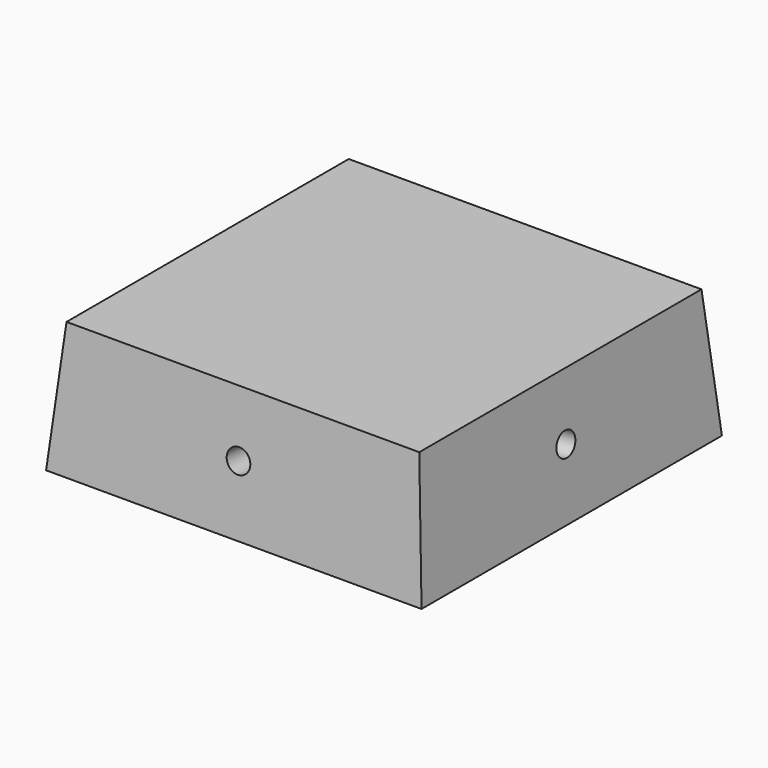
from build123d import *

# Parameters (mm, degrees)
F0_W        = 101.6
F0_H        = 101.6
F1_DEPTH    = 34.925
F2_T1_DEPTH = 299.3404177556
F2_T3_DEPTH = 299.3404177556
F3_R        = 3.175
F4_DEPTH    = 12.7
F5_R        = 3.175
F6_DEPTH    = 12.7
F7_R        = 3.175
F8_DEPTH    = 12.7
F9_R        = 3.175
F10_DEPTH   = 12.7
F11_W       = 75.6562831473
F11_H       = 25.4
F12_DEPTH   = 25.4
F13_SIZE2   = 25.39999
F13_SIZE    = 2.53999
F15_DEPTH   = 12.7
F16_R       = 2.54


# Not quite as in the source:
# - a fillet or chamfer that OpenCascade refuses, or shapes differently, is made with other operations: its cross-section is extruded or revolved along the edge and cut away or added
# - a fillet or chamfer is up to 0.001 mm smaller than in the source, because OpenCascade refuses the exact size


with BuildPart() as f1:
    # F0 (on Top) → F1 (new body)
    with BuildSketch(Plane.XY):
        Rectangle(F0_W, F0_H)
    extrude(amount=F1_DEPTH)

    # F2: chamfer of 3.3274 x 38.0323560322 on 4 edges, made by hand

    # F2_s2 → F2_t1 (cut)
    with BuildSketch(Plane.XZ.offset(-149.6702088778)):
        Polygon((-50.8, -3.1073560322), (-47.4726, 34.925), (-50.8, 34.925), align=None)
        Polygon((50.8, -3.1073560322), (47.4726, 34.925), (50.8, 34.925), align=None)
    extrude(amount=F2_T1_DEPTH, mode=Mode.SUBTRACT)

    # F2_s4 → F2_t3 (cut)
    with BuildSketch(Plane.YZ.offset(-149.6702088778)):
        Polygon((-50.8, -3.1073560322), (-47.4726, 34.925), (-50.8, 34.925), align=None)
        Polygon((50.8, -3.1073560322), (47.4726, 34.925), (50.8, 34.925), align=None)
    extrude(amount=F2_T3_DEPTH, mode=Mode.SUBTRACT)

    # F3 (on face) → F4 (cut)
    with BuildSketch(Plane(origin=(0, 50.1443235703, 4.3870598526), x_dir=(-1, 0, 0), z_dir=(0, 0.9961946981, 0.0871557427))):
        with Locations((0, 13.6719250414)):
            Circle(F3_R)
    extrude(amount=-F4_DEPTH, mode=Mode.SUBTRACT)

    # F5 (on face) → F6 (cut)
    with BuildSketch(Plane(origin=(0, -50.1443235703, 4.3870598526), x_dir=(1, 0, 0), z_dir=(0, -0.9961946981, 0.0871557427))):
        with Locations((0, 13.6719250414)):
            Circle(F5_R)
    extrude(amount=-F6_DEPTH, mode=Mode.SUBTRACT)

    # F7 (on face) → F8 (cut)
    with BuildSketch(Plane(origin=(50.1443235703, 0, 4.3870598526), x_dir=(0, 1, 0), z_dir=(0.9961946981, 0, 0.0871557427))):
        with Locations((0, 13.6719250414)):
            Circle(F7_R)
    extrude(amount=-F8_DEPTH, mode=Mode.SUBTRACT)

    # F9 (on face) → F10 (cut)
    with BuildSketch(Plane(origin=(-50.1443235703, 0, 4.3870598526), x_dir=(0, -1, 0), z_dir=(-0.9961946981, 0, 0.0871557427))):
        with Locations((0, 13.6719250414)):
            Circle(F9_R)
    extrude(amount=-F10_DEPTH, mode=Mode.SUBTRACT)

    # F11 (on face) → F12 (cut)
    with BuildSketch(Plane(origin=(0, 0, 0), x_dir=(1, 0, 0), z_dir=(0, 0, -1))):
        with Locations((0, -18.7781415736)):
            Rectangle(F11_W, F11_H)
    extrude(amount=-F12_DEPTH, mode=Mode.SUBTRACT)

    # F13 (size 2.54 and 25.4 in the source; OpenCascade refuses exactly that, so slightly less here)
    f13_edges = [f1.edges().sort_by_distance(p)[0] for p in [
        (0, 6.078142, 25.4),
        (-37.828142, 18.778142, 25.4),
        (0, 31.478142, 25.4),
        (37.828142, 18.778142, 25.4),
    ]]
    f13_side = f1.faces().sort_by_distance((0, 18.778142, 25.4))[0]
    chamfer(f13_edges, length=F13_SIZE, length2=F13_SIZE2, reference=f13_side)

    # F14 (on face) → F15 (cut)
    with BuildSketch(Plane(origin=(0, 0, 0), x_dir=(1, 0, 0), z_dir=(0, 0, -1))):
        with BuildLine():
            Line((-19.6998585016, 11.6611556837), (-10.5549017823, 11.6611556837))
            ThreePointArc((-10.5549017823, 11.6611556837), (-5.7924017823, 16.4236556837), (-10.5549017823, 21.1861556837))
            Line((-10.5549017823, 21.1861556837), (-19.6998585016, 21.1861556837))
            Line((-19.6998585016, 21.1861556837), (-25.4897605628, 21.1861556837))
            Line((-25.4897605628, 21.1861556837), (-25.4897605628, 11.6611556837))
            Line((-25.4897605628, 11.6611556837), (-25.4897605628, 5.814129021))
            Line((-25.4897605628, 5.814129021), (-19.6998585016, 5.814129021))
            Line((-19.6998585016, 5.814129021), (-19.6998585016, 11.6611556837))
        make_face()
        with BuildLine():
            Line((25.4897605628, 11.6611556837), (25.4897605628, 21.1861556837))
            Line((25.4897605628, 21.1861556837), (19.6998585016, 21.1861556837))
            Line((19.6998585016, 21.1861556837), (10.5549017823, 21.1861556837))
            ThreePointArc((10.5549017823, 21.1861556837), (5.7924017823, 16.4236556837), (10.5549017823, 11.6611556837))
            Line((10.5549017823, 11.6611556837), (19.6998585016, 11.6611556837))
            Line((19.6998585016, 11.6611556837), (19.6998585016, 5.814129021))
            Line((19.6998585016, 5.814129021), (25.4897605628, 5.814129021))
            Line((25.4897605628, 5.814129021), (25.4897605628, 11.6611556837))
        make_face()
    extrude(amount=-F15_DEPTH, mode=Mode.SUBTRACT)

    # F16
    f16_edges = [f1.edges().sort_by_distance(p)[0] for p in [
        (-15.12738, -11.661156, 12.7),
        (-5.792402, -16.423656, 12.7),
        (-18.022331, -21.186156, 12.7),
        (-25.489761, -13.500142, 12.7),
        (-22.59481, -5.814129, 12.7),
        (-19.699859, -8.737642, 12.7),
        (18.022331, -21.186156, 12.7),
        (5.792402, -16.423656, 12.7),
        (15.12738, -11.661156, 12.7),
        (19.699859, -8.737642, 12.7),
        (22.59481, -5.814129, 12.7),
        (25.489761, -13.500142, 12.7),
    ]]
    fillet(f16_edges, radius=F16_R)


solid = f1.part
